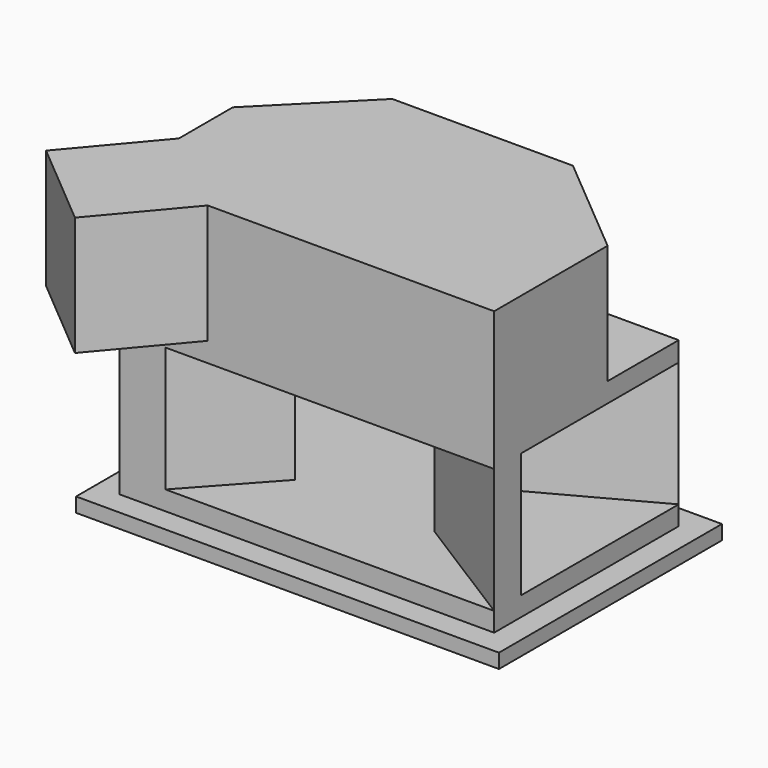
from build123d import *

# Parameters (mm, degrees)
F0_W      = 44
F0_H      = 29
F1_DEPTH  = 1.5
F2_W      = 39
F2_H      = 24
F3_DEPTH  = 15
F5_DEPTH  = 13
F8_W      = 24
F8_H      = 2.0449477285
F9_DEPTH  = 39
F11_DEPTH = 12.4
F12_W     = 12.0227243644
F12_H     = 12.4
F13_DEPTH = 11


# Not quite as in the source:
# - a feature names something its author has since deleted; it is built from what else it names


with BuildPart() as f1:
    # F0 (on Top) → F1 (new body)
    with BuildSketch(Plane.XY):
        with Locations((7.5298845768, 8.4944772368)):
            Rectangle(F0_W, F0_H)
    extrude(amount=F1_DEPTH)

    # F2 (on face) → F3 (join)
    with BuildSketch(Plane.XY.offset(1.5)):
        with Locations((7.5298845768, 8.4944772368)):
            Rectangle(F2_W, F2_H)
    extrude(amount=F3_DEPTH)

    # F4 (on face) → F5 (cut)
    with BuildSketch(Plane.XY.offset(16.5)):
        Polygon((22.4261898547, 20.4944772368), (-11.9701154232, 20.4944772368), (-11.9701154232, -3.5055227632), (0, 4.4034305029), (-7.16903992, -3.5055227632), (27.0298845768, -3.5055227632), (14.4714023918, 4.4034305029), (27.0298845768, 0), (27.0298845768, 20.4944772368), (14.4714023918, 13.7267839164), align=None)
    extrude(amount=-F5_DEPTH, mode=Mode.SUBTRACT)

    # F8 (on face) → F9 (join)
    with BuildSketch(Plane(origin=(-11.9701154232, 0, 0), x_dir=(0, -1, 0), z_dir=(-1, 0, 0))):
        with Locations((-8.4944772368, 17.5224738643)):
            Rectangle(F8_W, F8_H)
    extrude(amount=-F9_DEPTH)

    # F10 (on face) → F11 (join)
    with BuildSketch(Plane.XY.offset(18.5449477285)):
        Polygon((16.0282067955, 20.4944772368), (-2.7732178569, 20.4944772368), (-11.9701154232, 11.2487543374), (-11.9701154232, 4.2380536906), (-2.7732178569, -3.5055227632), (27.0298845768, -3.5055227632), (27.0298845768, 11.2487543374), align=None)
    extrude(amount=F11_DEPTH)

    # F12 (on face) → F13 (join)
    with BuildSketch(Plane(origin=(-2.8775827287, -3.4176499389, 0), x_dir=(0.7649595289, -0.6440783486, 0), z_dir=(-0.6440783486, -0.7649595289, 0))):
        with Locations((-5.8749302955, 24.7449477285)):
            Rectangle(F12_W, F12_H)
    extrude(amount=F13_DEPTH)


solid = f1.part
